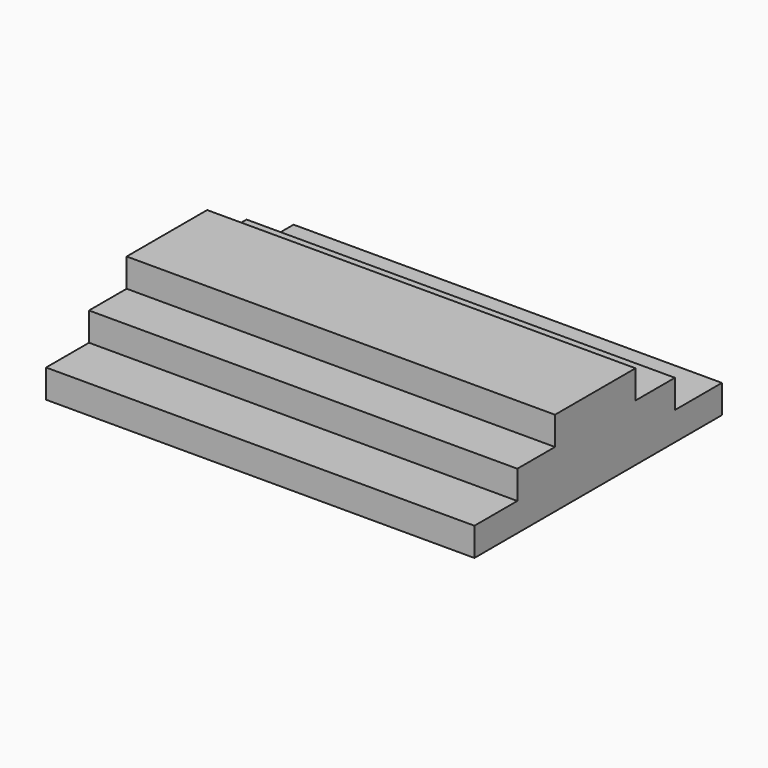
from build123d import *

# Parameters (mm, degrees)
F0_W     = 76.6426213086
F0_H     = 55.3530044854
F1_DEPTH = 25.4
F2_W     = 76.6426213086
F2_H     = 9.5973666757
F3_DEPTH = 20.32
F2_H_2   = 8.4236329421
F4_DEPTH = 15.24
F2_H_3   = 9.6555026248
F5_DEPTH = 10.16
F2_H_4   = 8.3485189825
F6_DEPTH = 10.16
F2_H_5   = 8.8109364733
F7_DEPTH = 15.24
F2_H_6   = 10.5170467868
F8_DEPTH = 20.32


with BuildPart() as f1:
    # F0 (on Top) → F1 (new body)
    with BuildSketch(Plane.XY):
        with Locations((-0.0834930688, -1.8811021)):
            Rectangle(F0_W, F0_H)
    extrude(amount=F1_DEPTH)

    # F2 (on face) → F3 (cut)
    with BuildSketch(Plane.XY.offset(25.4)):
        with Locations((-0.0834930688, -24.7589210048)):
            Rectangle(F2_W, F2_H)
    extrude(amount=-F3_DEPTH, mode=Mode.SUBTRACT)

    # F2 (on face) → F4 (cut)
    with BuildSketch(Plane.XY.offset(25.4)):
        with Locations((-0.0834930688, -15.7484211959)):
            Rectangle(F2_W, F2_H_2)
    extrude(amount=-F4_DEPTH, mode=Mode.SUBTRACT)

    # F2 (on face) → F5 (cut)
    with BuildSketch(Plane.XY.offset(25.4)):
        with Locations((-0.0834930688, -6.7088534124)):
            Rectangle(F2_W, F2_H_3)
    extrude(amount=-F5_DEPTH, mode=Mode.SUBTRACT)

    # F2 (on face) → F6 (cut)
    with BuildSketch(Plane.XY.offset(25.4)):
        with Locations((-0.0834930688, 2.2931573913)):
            Rectangle(F2_W, F2_H_4)
    extrude(amount=-F6_DEPTH, mode=Mode.SUBTRACT)

    # F2 (on face) → F7 (cut)
    with BuildSketch(Plane.XY.offset(25.4)):
        with Locations((-0.0834930688, 10.8728851192)):
            Rectangle(F2_W, F2_H_5)
    extrude(amount=-F7_DEPTH, mode=Mode.SUBTRACT)

    # F2 (on face) → F8 (cut)
    with BuildSketch(Plane.XY.offset(25.4)):
        with Locations((-0.0834930688, 20.5368767492)):
            Rectangle(F2_W, F2_H_6)
    extrude(amount=-F8_DEPTH, mode=Mode.SUBTRACT)


solid = f1.part
